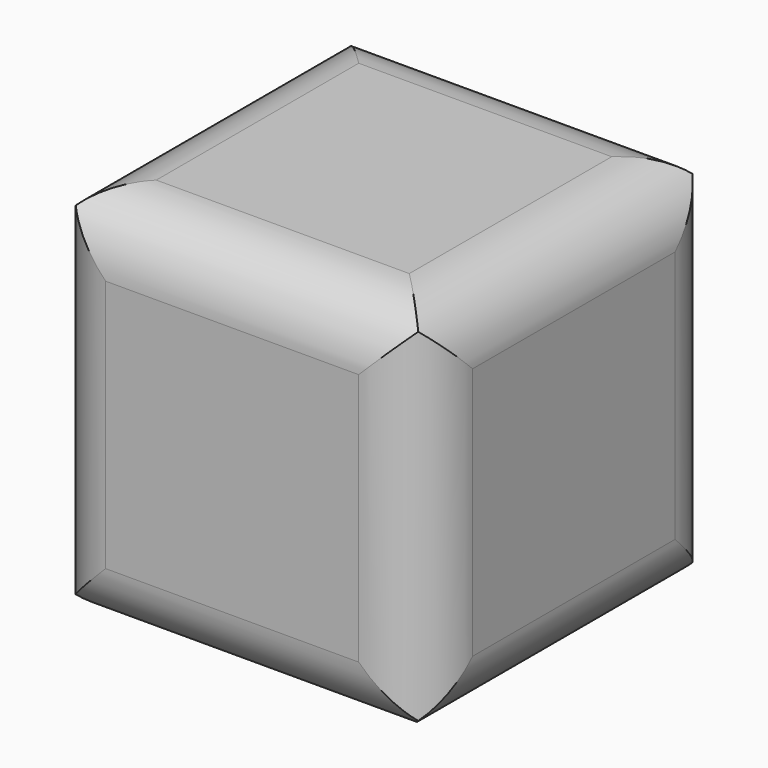
from build123d import *

# Parameters (mm, degrees)
F0_W        = 30
F0_H        = 30
F1_DEPTH    = 30
F2_R        = 5
F3_T1_DEPTH = 50
F3_T3_DEPTH = 55
F4_T1_DEPTH = 50
F4_T3_DEPTH = 55
F6_T1_DEPTH = 45


# Not quite as in the source:
# - a fillet or chamfer that OpenCascade refuses, or shapes differently, is made with other operations: its cross-section is extruded or revolved along the edge and cut away or added
# - a feature of the source that left no trace in its solid (it failed there, or was rolled back) is left out


with BuildPart() as f1:
    # F0 (on Right) → F1 (new body)
    with BuildSketch(Plane.YZ):
        with Locations((-5.478883007, 2.1195821464)):
            Rectangle(F0_W, F0_H)
    extrude(amount=F1_DEPTH)

    # F2
    f2_edges = [f1.edges().sort_by_distance(p)[0] for p in [
        (30, -5.478883, -12.880418),
        (30, 9.521117, 2.119582),
        (30, -5.478883, 17.119582),
        (30, -20.478883, 2.119582),
    ]]
    fillet(f2_edges, radius=F2_R)

    # F3: fillet of radius 5 on 4 edges, made by hand

    # F3_s2 → F3_t1 (cut)
    with BuildSketch(Plane.YZ.offset(-12.5)):
        with BuildLine():
            ThreePointArc((4.521116993, -12.8804178536), (8.0566508989, -11.4159517595), (9.521116993, -7.8804178536))
            Line((9.521116993, -7.8804178536), (9.521116993, -12.8804178536))
            Line((9.521116993, -12.8804178536), (4.521116993, -12.8804178536))
        make_face()
        with BuildLine():
            ThreePointArc((9.521116993, 12.1195821464), (8.0566508989, 15.6551160523), (4.521116993, 17.1195821464))
            Line((4.521116993, 17.1195821464), (9.521116993, 17.1195821464))
            Line((9.521116993, 17.1195821464), (9.521116993, 12.1195821464))
        make_face()
    extrude(amount=F3_T1_DEPTH, mode=Mode.SUBTRACT)

    # F3_s4 → F3_t3 (cut)
    with BuildSketch(Plane.XY.offset(-25.3804178536)):
        with BuildLine():
            ThreePointArc((0, 4.521116993), (1.4644660941, 8.0566508989), (5, 9.521116993))
            Line((5, 9.521116993), (0, 9.521116993))
            Line((0, 9.521116993), (0, 4.521116993))
        make_face()
    extrude(amount=F3_T3_DEPTH, mode=Mode.SUBTRACT)

    # F4: fillet of radius 5 on 4 edges, made by hand

    # F4_s2 → F4_t1 (cut)
    with BuildSketch(Plane.YZ.offset(-12.5)):
        with BuildLine():
            ThreePointArc((-20.478883007, 12.1195821464), (-19.0144169129, 15.6551160523), (-15.478883007, 17.1195821464))
            Line((-15.478883007, 17.1195821464), (-20.478883007, 17.1195821464))
            Line((-20.478883007, 17.1195821464), (-20.478883007, 12.1195821464))
        make_face()
        with BuildLine():
            ThreePointArc((-15.478883007, -12.8804178536), (-19.0144169129, -11.4159517595), (-20.478883007, -7.8804178536))
            Line((-20.478883007, -7.8804178536), (-20.478883007, -12.8804178536))
            Line((-20.478883007, -12.8804178536), (-15.478883007, -12.8804178536))
        make_face()
    extrude(amount=F4_T1_DEPTH, mode=Mode.SUBTRACT)

    # F4_s4 → F4_t3 (cut)
    with BuildSketch(Plane.XY.offset(-25.3804178536)):
        with BuildLine():
            ThreePointArc((5, -20.478883007), (1.4644660941, -19.0144169129), (0, -15.478883007))
            Line((0, -15.478883007), (0, -20.478883007))
            Line((0, -20.478883007), (5, -20.478883007))
        make_face()
    extrude(amount=F4_T3_DEPTH, mode=Mode.SUBTRACT)

    # F6: fillet of radius 5 on 4 edges, made by hand

    # F6_s2 → F6_t1 (cut)
    with BuildSketch(Plane.XZ.offset(-17.021116993)):
        with BuildLine():
            ThreePointArc((5, -12.8804178536), (1.4644660941, -11.4159517595), (0, -7.8804178536))
            Line((0, -7.8804178536), (0, -12.8804178536))
            Line((0, -12.8804178536), (5, -12.8804178536))
        make_face()
        with BuildLine():
            ThreePointArc((0, 12.1195821464), (1.4644660941, 15.6551160523), (5, 17.1195821464))
            Line((5, 17.1195821464), (0, 17.1195821464))
            Line((0, 17.1195821464), (0, 12.1195821464))
        make_face()
    extrude(amount=F6_T1_DEPTH, mode=Mode.SUBTRACT)


solid = f1.part
